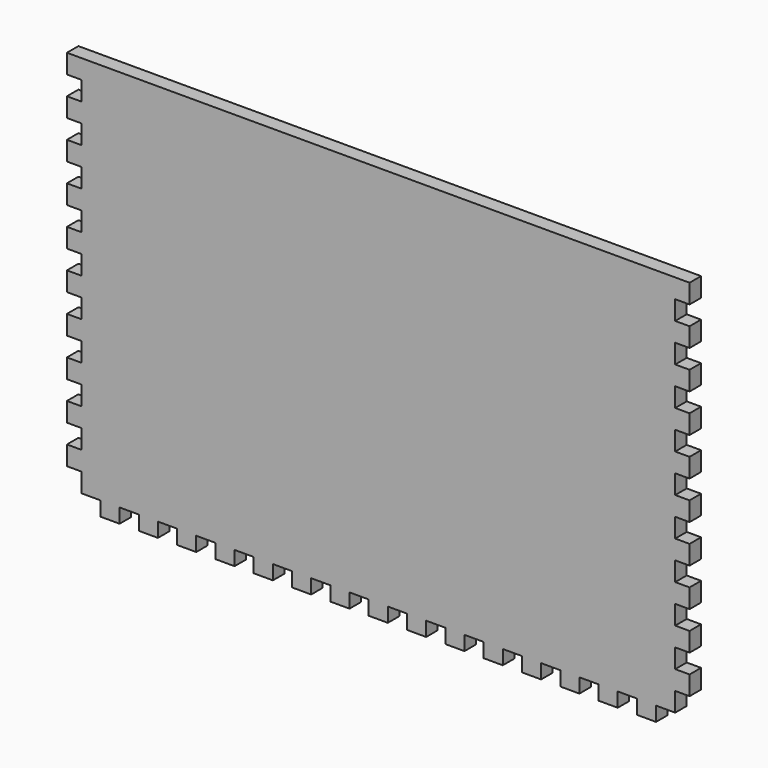
from build123d import *

# Parameters (mm, degrees)
F0_W     = 372
F0_H     = 240
F1_DEPTH = 9
F2_W     = 9
F2_H     = 12
F3_DEPTH = 9
F4_W     = 12
F4_H     = 9
F5_DEPTH = 9


with BuildPart() as f1:
    # F0 (on Front) → F1 (new body)
    with BuildSketch(Plane.XZ):
        Rectangle(F0_W, F0_H)
    extrude(amount=F1_DEPTH)

    # F2 (on face) → F3 (join, through all)
    with BuildSketch(Plane.XZ.offset(9)):
        with Locations((-190.5, 114)):
            Rectangle(F2_W, F2_H)
        with Locations((-190.5, 90)):
            Rectangle(F2_W, F2_H)
        with Locations((-190.5, 66)):
            Rectangle(F2_W, F2_H)
        with Locations((-190.5, 42)):
            Rectangle(F2_W, F2_H)
        with Locations((-190.5, 18)):
            Rectangle(F2_W, F2_H)
        with Locations((-190.5, -6)):
            Rectangle(F2_W, F2_H)
        with Locations((-190.5, -30)):
            Rectangle(F2_W, F2_H)
        with Locations((-190.5, -54)):
            Rectangle(F2_W, F2_H)
        with Locations((-190.5, -78)):
            Rectangle(F2_W, F2_H)
        with Locations((-190.5, -102)):
            Rectangle(F2_W, F2_H)
        with Locations((190.5, 114)):
            Rectangle(F2_W, F2_H)
        with Locations((190.5, 90)):
            Rectangle(F2_W, F2_H)
        with Locations((190.5, -30)):
            Rectangle(F2_W, F2_H)
        with Locations((190.5, -102)):
            Rectangle(F2_W, F2_H)
        with Locations((190.5, -6)):
            Rectangle(F2_W, F2_H)
        with Locations((190.5, -54)):
            Rectangle(F2_W, F2_H)
        with Locations((190.5, -78)):
            Rectangle(F2_W, F2_H)
        with Locations((190.5, 18)):
            Rectangle(F2_W, F2_H)
        with Locations((190.5, 42)):
            Rectangle(F2_W, F2_H)
        with Locations((190.5, 66)):
            Rectangle(F2_W, F2_H)
    extrude(amount=-F3_DEPTH)

    # F4 (on face) → F5 (join, through all)
    with BuildSketch(Plane.XZ.offset(9)):
        with Locations((0, -124.5)):
            Rectangle(F4_W, F4_H)
        with Locations((24, -124.5)):
            Rectangle(F4_W, F4_H)
        with Locations((48, -124.5)):
            Rectangle(F4_W, F4_H)
        with Locations((72, -124.5)):
            Rectangle(F4_W, F4_H)
        with Locations((96, -124.5)):
            Rectangle(F4_W, F4_H)
        with Locations((120, -124.5)):
            Rectangle(F4_W, F4_H)
        with Locations((144, -124.5)):
            Rectangle(F4_W, F4_H)
        with Locations((168, -124.5)):
            Rectangle(F4_W, F4_H)
        with Locations((-24, -124.5)):
            Rectangle(F4_W, F4_H)
        with Locations((-96, -124.5)):
            Rectangle(F4_W, F4_H)
        with Locations((-120, -124.5)):
            Rectangle(F4_W, F4_H)
        with Locations((-168, -124.5)):
            Rectangle(F4_W, F4_H)
        with Locations((-48, -124.5)):
            Rectangle(F4_W, F4_H)
        with Locations((-144, -124.5)):
            Rectangle(F4_W, F4_H)
        with Locations((-72, -124.5)):
            Rectangle(F4_W, F4_H)
    extrude(amount=-F5_DEPTH)


solid = f1.part
